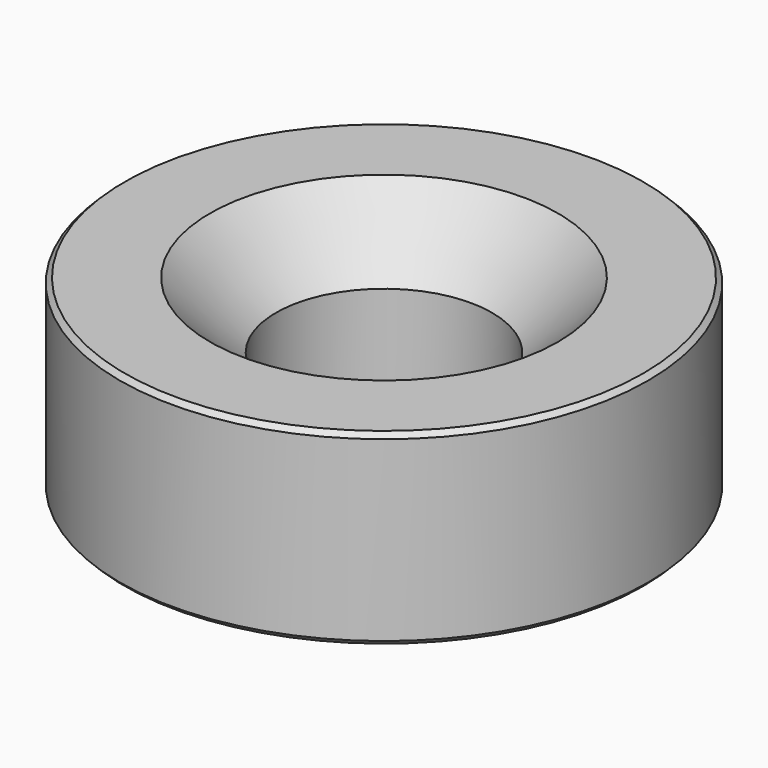
from build123d import *

# Parameters (mm, degrees)
F0_R     = 11
F0_R_2   = 4.5
F1_DEPTH = 7.8
F2_SIZE  = 0.2
F3_SIZE  = 2.75


with BuildPart() as f1:
    # F0 (on Top) → F1 (new body)
    with BuildSketch(Plane.XY):
        Circle(F0_R)
        Circle(F0_R_2, mode=Mode.SUBTRACT)
    extrude(amount=F1_DEPTH)

    # F2
    f2_edges = [f1.edges().sort_by_distance(p)[0] for p in [
        (-11, 0, 7.8),
        (-11, 0, 0),
        (-4.5, 0, 0),
    ]]
    chamfer(f2_edges, length=F2_SIZE)

    # F3
    f3_edges = [f1.edges().sort_by_distance(p)[0] for p in [
        (-4.5, 0, 7.8),
    ]]
    chamfer(f3_edges, length=F3_SIZE)


solid = f1.part
